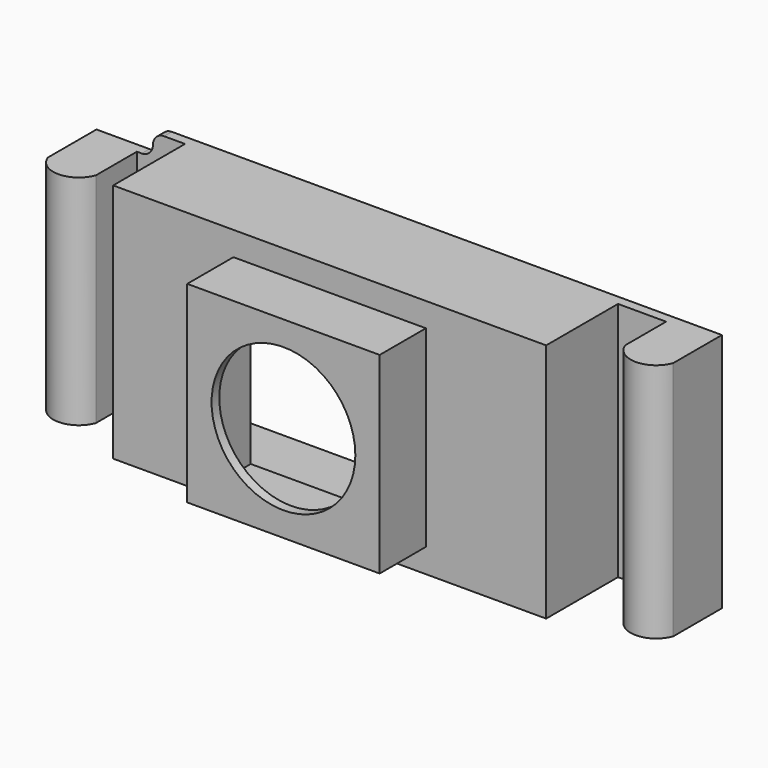
from build123d import *

# Parameters (mm, degrees)
F0_W      = 60
F0_H      = 60
F0_R      = 22.4096796893
F1_DEPTH  = 3
F2_W      = 60
F2_H      = 60
F2_W_2    = 54
F2_H_2    = 54
F3_DEPTH  = 15
F4_W      = 135
F4_H      = 75
F4_W_2    = 54
F4_H_2    = 54
F5_DEPTH  = 3
F6_W      = 135
F6_H      = 75
F6_W_2    = 129
F6_H_2    = 69
F7_DEPTH  = 25
F8_W      = 195
F8_H      = 75
F8_W_2    = 129
F8_H_2    = 69
F9_DEPTH  = 3
F10_W     = 15
F10_H     = 68
F11_DEPTH = 25
F12_W     = 15
F12_H     = 75
F13_DEPTH = 25
F15_DEPTH = 200
F17_DEPTH = 25
F18_R     = 3.49999
F21_DEPTH = 60


# Not quite as in the source:
# - a fillet or chamfer is up to 0.001 mm smaller than in the source, because OpenCascade refuses the exact size


with BuildPart() as f1:
    # F0 (on Front) → F1 (new body)
    with BuildSketch(Plane.XZ):
        Rectangle(F0_W, F0_H)
        Circle(F0_R, mode=Mode.SUBTRACT)
    extrude(amount=F1_DEPTH)

    # F2 (on face) → F3 (join)
    with BuildSketch(Plane(origin=(0, 0, 0), x_dir=(-1, 0, 0), z_dir=(0, 1, 0))):
        Rectangle(F2_W, F2_H)
        Rectangle(F2_W_2, F2_H_2, mode=Mode.SUBTRACT)
    extrude(amount=F3_DEPTH)

    # F4 (on face) → F5 (join)
    with BuildSketch(Plane(origin=(0, 15, 0), x_dir=(-1, 0, 0), z_dir=(0, 1, 0))):
        Rectangle(F4_W, F4_H)
        Rectangle(F4_W_2, F4_H_2, mode=Mode.SUBTRACT)
    extrude(amount=F5_DEPTH)

    # F6 (on face) → F7 (join)
    with BuildSketch(Plane(origin=(0, 18, 0), x_dir=(-1, 0, 0), z_dir=(0, 1, 0))):
        Rectangle(F6_W, F6_H)
        Rectangle(F6_W_2, F6_H_2, mode=Mode.SUBTRACT)
    extrude(amount=F7_DEPTH)

    # F8 (on face) → F9 (join)
    with BuildSketch(Plane(origin=(0, 43, 0), x_dir=(-1, 0, 0), z_dir=(0, 1, 0))):
        Rectangle(F8_W, F8_H)
        Rectangle(F8_W_2, F8_H_2, mode=Mode.SUBTRACT)
    extrude(amount=F9_DEPTH)

    # F10 (on face) → F11 (join)
    with BuildSketch(Plane.XZ.offset(-43)):
        with Locations((-90, -3.5)):
            Rectangle(F10_W, F10_H)
    extrude(amount=F11_DEPTH)

    # F12 (on face) → F13 (join)
    with BuildSketch(Plane.XZ.offset(-43)):
        with Locations((90, 0)):
            Rectangle(F12_W, F12_H)
    extrude(amount=F13_DEPTH)

    # F14 (on face) → F15 (cut)
    with BuildSketch(Plane.XY.offset(37.5)):
        with BuildLine():
            ThreePointArc((-82.5, 27), (-90, 21.7838821814), (-97.5, 27))
            Line((-97.5, 27), (-97.5, 18))
            Line((-97.5, 18), (-82.5, 18))
            Line((-82.5, 18), (-82.5, 27))
        make_face()
        with BuildLine():
            ThreePointArc((97.5, 27), (90, 21.7838821814), (82.5, 27))
            Line((82.5, 27), (82.5, 18))
            Line((82.5, 18), (97.5, 18))
            Line((97.5, 18), (97.5, 27))
        make_face()
    extrude(amount=-F15_DEPTH, mode=Mode.SUBTRACT)

    # F16 (on face) → F17 (cut)
    with BuildSketch(Plane.XZ.offset(-43)):
        Polygon((-77.5, 37.5), (-82.5, 37.5), (-97.5, 37.5), (-97.5, 30.5), (-82.5, 30.5), (-77.5, 30.5), align=None)
    extrude(amount=-F17_DEPTH, mode=Mode.SUBTRACT)

    # F18 (radius 3.5 in the source; OpenCascade refuses exactly that, so slightly less here)
    f18_edges = [f1.edges().sort_by_distance(p)[0] for p in [
        (-77.5, 44.5, 30.5),
        (-77.5, 44.5, 37.5),
    ]]
    fillet(f18_edges, radius=F18_R)

    # F20 (on face) → F21 (cut)
    with BuildSketch(Plane.XY.offset(30)):
        Polygon((-30, -3), (-50, 15), (-50, -3), align=None)
    extrude(amount=-F21_DEPTH, mode=Mode.SUBTRACT)


solid = f1.part
